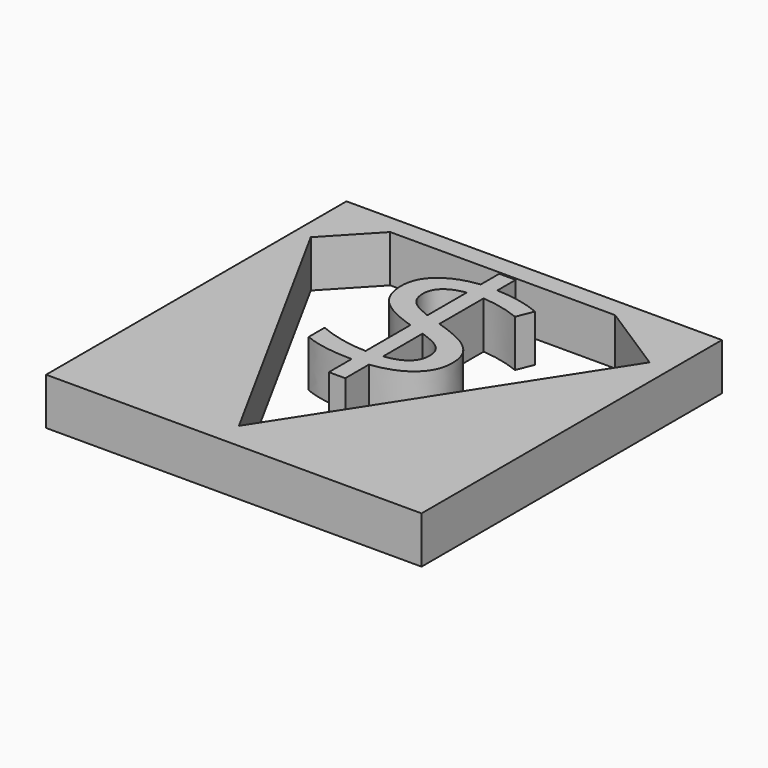
from build123d import *

# Parameters (mm, degrees)
F0_W         = 50.8
F0_H         = 50.8
F0_TEXT_SIZE = 35.2777777778
F1_DEPTH     = 6.35


# Not quite as in the source:
# - Text() gives the source's letters only with a copy of the font that has no kerning and outlines rounded to 1/6400 em; it was checked with that copy


with BuildPart() as f1:
    # F0 (on Top) → F1 (new body)
    with BuildSketch(Plane.XY):
        with Locations((25.4, 25.4)):
            Rectangle(F0_W, F0_H)
        Polygon((2.1865079179, 42.0295447111), (8.0005861417, 48.1959916651), (38.4379364952, 48.1959916651), (48.0221933685, 42.0295447111), (23.2192613184, 3.5932111047), align=None, mode=Mode.SUBTRACT)
        with Locations((14.0098454431, 21.1645231307)):
            Text('$', F0_TEXT_SIZE, font='Open Sans', text_align=(TextAlign.LEFT, TextAlign.BOTTOM))
    extrude(amount=F1_DEPTH)


solid = f1.part
